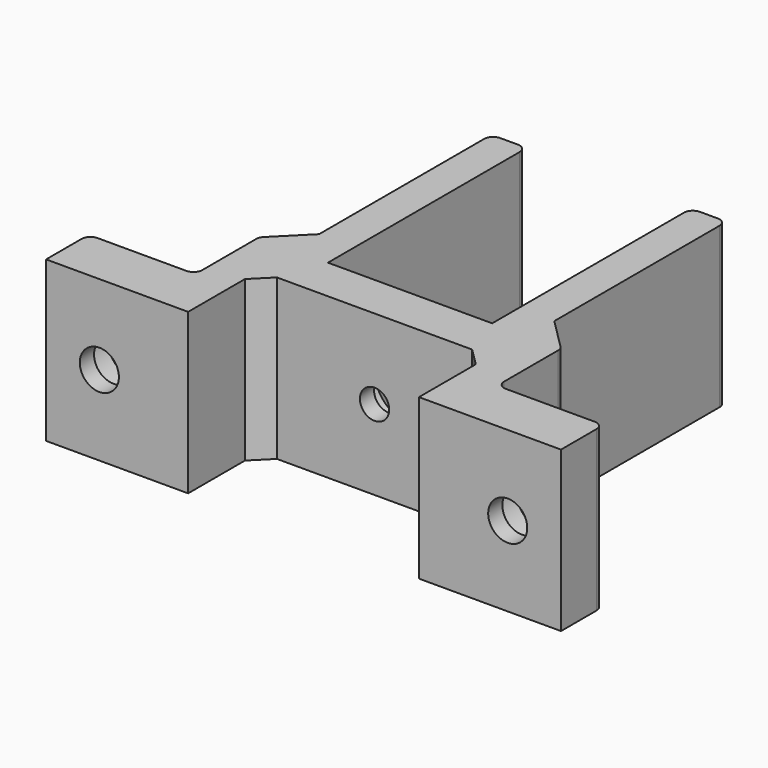
from build123d import *

# Parameters (mm, degrees)
F1_DEPTH             = 18
F4_D                 = 4.4
F4_CBORE_D           = 8.25
F4_CBORE_DEPTH       = 4
F4_ON_F3_D           = 4.4
F4_ON_F3_CBORE_D     = 8.25
F4_ON_F3_CBORE_DEPTH = 4
F5_SIZE              = 2
F6_R                 = 1
F7_R                 = 1.65
F8_DEPTH             = 15.001
F9_R                 = 4
F10_DEPTH            = 3


with BuildPart() as f1:
    # F0 (on Top) → F1 (new body)
    with BuildSketch(Plane.XY):
        Polygon((0, 6), (0, 0), (16, 0), (16, 10), (42, 10), (42, 0), (58, 0), (58, 6), (46, 6), (46, 15), (42.25, 18.75), (42.25, 43), (38.25, 43), (38.25, 15), (19.75, 15), (19.75, 43), (15.75, 43), (15.75, 18.75), (12, 15), (12, 6), align=None)
    extrude(amount=F1_DEPTH)

    # F4 (through all)
    with Locations(Plane(origin=(0, 6, 0), x_dir=(-1, 0, 0), z_dir=(0, 1, 0))):
        with Locations((-52, 9)):
            CounterBoreHole(F4_D / 2, F4_CBORE_D / 2, F4_CBORE_DEPTH)

    # F4 on F3 (through all)
    with Locations(Plane(origin=(0, 6, 0), x_dir=(-1, 0, 0), z_dir=(0, 1, 0))):
        with Locations((-6, 9)):
            CounterBoreHole(F4_ON_F3_D / 2, F4_ON_F3_CBORE_D / 2, F4_ON_F3_CBORE_DEPTH)

    # F5
    f5_edges = [f1.edges().sort_by_distance(p)[0] for p in [
        (16, 10, 9),
        (42, 10, 9),
    ]]
    chamfer(f5_edges, length=F5_SIZE)

    # F6
    f6_edges = [f1.edges().sort_by_distance(p)[0] for p in [
        (46, 6, 9),
        (38.25, 43, 9),
        (19.75, 43, 9),
        (12, 6, 9),
        (0, 6, 9),
        (58, 6, 9),
        (12, 15, 9),
        (15.75, 43, 9),
        (46, 15, 9),
        (42.25, 43, 9),
    ]]
    fillet(f6_edges, radius=F6_R)

    # F7 (on face) → F8 (cut, through all)
    with BuildSketch(Plane(origin=(0, 15, 0), x_dir=(-1, 0, 0), z_dir=(0, 1, 0))):
        with Locations((-29, 9)):
            Circle(F7_R)
    extrude(amount=-F8_DEPTH, mode=Mode.SUBTRACT)

    # F9 (on face) → F10 (cut)
    with BuildSketch(Plane(origin=(0, 15, 0), x_dir=(-1, 0, 0), z_dir=(0, 1, 0))):
        with Locations((-29, 9)):
            Circle(F9_R)
    extrude(amount=-F10_DEPTH, mode=Mode.SUBTRACT)


solid = f1.part
